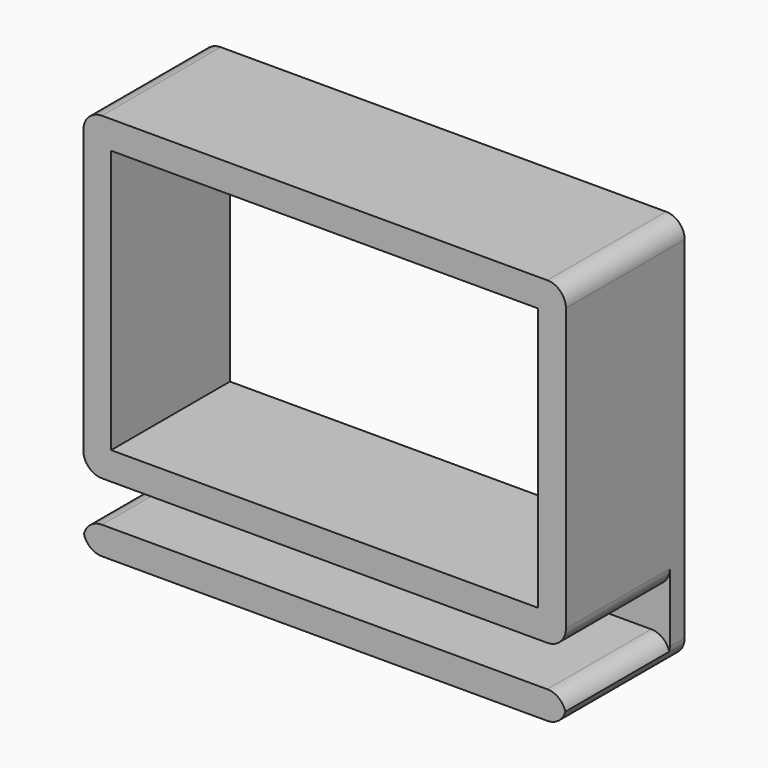
from build123d import *

# Parameters (mm, degrees)
F0_W     = 26
F0_H     = 17.2
F0_W_2   = 23
F0_H_2   = 14.2
F1_DEPTH = 8
F0_H_3   = 1.5
F2_W     = 26
F2_H     = 5.2
F3_DEPTH = 1
F4_F1_R  = 1
F4_F2_R  = 1
F4_F3_R  = 1
F4_F4_R  = 1
F4_F5_R  = 1
F4_F6_R  = 1
F4_F7_R  = 1
F4_F8_R  = 1


with BuildPart() as f1:
    # F0 (on Front) → F1 (new body)
    with BuildSketch(Plane.XZ):
        Rectangle(F0_W, F0_H)
        Rectangle(F0_W_2, F0_H_2, mode=Mode.SUBTRACT)
    extrude(amount=F1_DEPTH)



with BuildPart() as f1b:
    # F0 (on Front) → F1, piece 2 (new body)
    with BuildSketch(Plane.XZ):
        with Locations((0, -11.55)):
            Rectangle(F0_W, F0_H_3)
    extrude(amount=F1_DEPTH)


with BuildPart() as f1_1:
    add(f1.part)

    add(f1b.part)  # F3 merges F1b
    # F2 (on face) → F3 (join)
    with BuildSketch(Plane(origin=(0, 0, 0), x_dir=(-1, 0, 0), z_dir=(0, 1, 0))):
        with Locations((0, -9.7)):
            Rectangle(F2_W, F2_H)
    extrude(amount=-F3_DEPTH)

    # F4: fillet of radius 1 on 8 edges, made by hand

    # F4_f1
    f4_f1_edges = [f1_1.edges().sort_by_distance(p)[0] for p in [
        (13, -4.5, -8.6),
    ]]
    fillet(f4_f1_edges, radius=F4_F1_R)

    # F4_f2
    f4_f2_edges = [f1_1.edges().sort_by_distance(p)[0] for p in [
        (-13, -4.5, -8.6),
    ]]
    fillet(f4_f2_edges, radius=F4_F2_R)

    # F4_f3
    f4_f3_edges = [f1_1.edges().sort_by_distance(p)[0] for p in [
        (-13, -4.5, -10.8),
    ]]
    fillet(f4_f3_edges, radius=F4_F3_R)

    # F4_f4
    f4_f4_edges = [f1_1.edges().sort_by_distance(p)[0] for p in [
        (13, -4.5, -10.8),
    ]]
    fillet(f4_f4_edges, radius=F4_F4_R)

    # F4_f5
    f4_f5_edges = [f1_1.edges().sort_by_distance(p)[0] for p in [
        (13, -4, 8.6),
    ]]
    fillet(f4_f5_edges, radius=F4_F5_R)

    # F4_f6
    f4_f6_edges = [f1_1.edges().sort_by_distance(p)[0] for p in [
        (-13, -4, 8.6),
    ]]
    fillet(f4_f6_edges, radius=F4_F6_R)

    # F4_f7
    f4_f7_edges = [f1_1.edges().sort_by_distance(p)[0] for p in [
        (13, -4, -12.3),
    ]]
    fillet(f4_f7_edges, radius=F4_F7_R)

    # F4_f8
    f4_f8_edges = [f1_1.edges().sort_by_distance(p)[0] for p in [
        (-13, -4, -12.3),
    ]]
    fillet(f4_f8_edges, radius=F4_F8_R)


solid = f1_1.part
